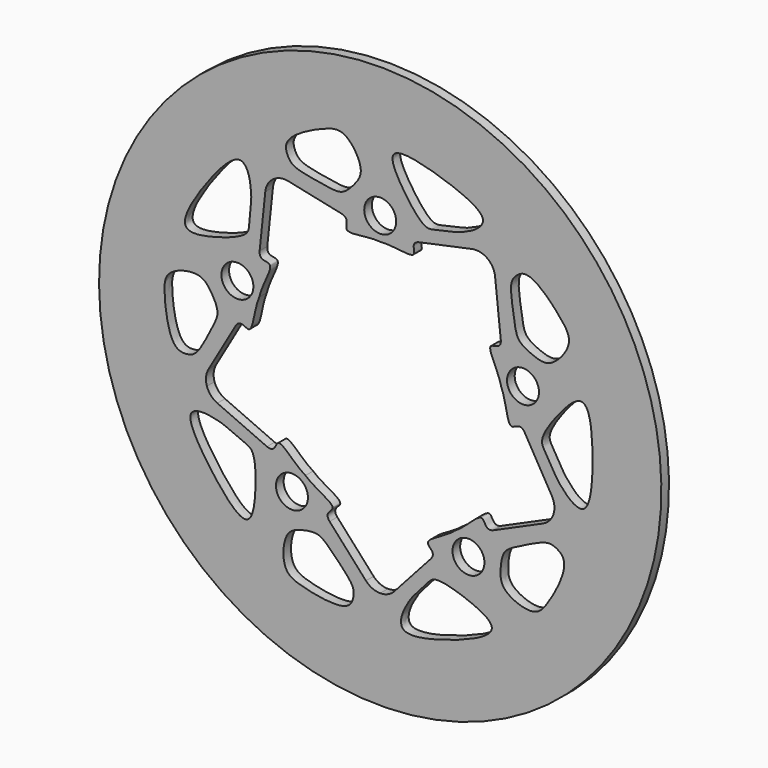
from build123d import *

# Parameters (mm, degrees)
F1_DEPTH = 3
F3_DEPTH = 3.001
F5_COUNT = 5


# Not quite as in the source:
# - a feature names something its author has since deleted; it is built from what else it names


with BuildPart() as f1:
    # F0 (on Front) → F1 (new body)
    with BuildSketch(Plane.XZ):
        with BuildLine():
            Line((0, 0), (51.7251022017, 71.193495505))
            ThreePointArc((51.7251022017, 71.193495505), (0, 88), (-51.7251022017, 71.193495505))
            Line((-51.7251022017, 71.193495505), (0, 0))
        make_face()
    extrude(amount=F1_DEPTH)

    # F2 (on face) → F3 (cut, through all)
    with BuildSketch(Plane.XZ.offset(3)):
        with BuildLine():
            ThreePointArc((0, 42), (5, 47), (0, 52))
            ThreePointArc((0, 52), (-5, 47), (0, 42))
        make_face()
        with BuildLine():
            ThreePointArc((35.9636588543, 41.9138488829), (33.5232389959, 46.1407800695), (28.7490573372, 47.1555637077))
            Line((28.7490573372, 47.1555637077), (12.1205481247, 43.6210649638))
            add(Edge.make_bspline(
                [(0, 39.7937037051), (4.2587816715, 40.1929393411), (13.3803774655, 37.3030713655), (9.4487516397, 42.9875629744), (12.1205481247, 43.6210649638)],
                knots=[0, 0, 0, 0, 0.6175220628, 1, 1, 1, 1], degree=3))
            add(Edge.make_bspline(
                [(0, 39.7937037051), (-4.2587816715, 40.1929393411), (-13.3803774655, 37.3030713655), (-9.4487516397, 42.9875629744), (-12.1205481247, 43.6210649638)],
                knots=[0, 0, 0, 0, 0.6175220628, 1, 1, 1, 1], degree=3))
            Line((-12.1205481247, 43.6210649638), (-28.7490573372, 47.1555637077))
            ThreePointArc((-28.7490573372, 47.1555637077), (-33.5232389959, 46.1407800695), (-35.9636588543, 41.9138488829))
            Line((-35.9636588543, 41.9138488829), (-2.9421695508, -4.9399328418))
            Line((-2.9421695508, -4.9399328418), (12.7777997404, -4.9399328418))
            Line((12.7777997404, -4.9399328418), (35.9636588543, 41.9138488829))
        make_face()
        with BuildLine():
            add(Edge.make_bspline(
                [(-28.5915061831, 53.4918643534), (-28.0674536128, 52.6606457363), (-26.5174759631, 51.2570025021), (-19.4438074989, 50.1029196457), (-14.2533650642, 49.1722397117), (-11.1439460512, 49.5979391514), (-7.4521347596, 53.4948210478), (-4.7909060568, 58.0275481358), (-10.6706291595, 67.3062899705), (-17.3590306737, 65.5999393826), (-25.9414121965, 61.562331704), (-30.2648454395, 57.2735760645), (-29.171944739, 54.4125188088), (-28.5915061831, 53.4918643534)],
                knots=[0, 0, 0, 0, 0.0658419042, 0.1698464289, 0.2604897957, 0.3264810991, 0.4143446925, 0.5005467885, 0.6178182582, 0.7140387999, 0.8360790262, 0.9270737671, 1, 1, 1, 1], degree=3))
        make_face()
        with BuildLine():
            add(Edge.make_bspline(
                [(4.2171571404, 65.2592182159), (2.934068333, 63.5341672141), (7.7043281913, 55.1663980521), (13.8126235602, 47.727511354), (16.9974975366, 48.7045519565), (19.4278683832, 49.1682997699), (21.6974179791, 49.751798731), (24.2393332206, 50.2035724255), (27.1518145661, 51.4103491912), (30.6429989505, 53.1324679062), (34.2219239988, 57.8113404446), (19.7511153655, 64.1504125332), (5.7809723565, 67.3616923313), (4.2171571404, 65.2592182159)],
                knots=[0, 0, 0, 0, 0.1229386585, 0.2430861429, 0.3051746062, 0.3653848965, 0.4241190304, 0.4854014571, 0.5534869806, 0.6309447575, 0.7032321985, 0.850163649, 1, 1, 1, 1], degree=3))
        make_face()
    extrude(amount=-F3_DEPTH, mode=Mode.SUBTRACT)

    # F5: F1 ×5 about axis
    f5_axis = Axis((0, -38.883369416, 0), (0, -1, 0))


with BuildPart() as f1_1:
    add(f1.part)
    for i in range(1, F5_COUNT):
        add(f1.part.rotate(f5_axis, i * 360 / F5_COUNT))


solid = f1_1.part
